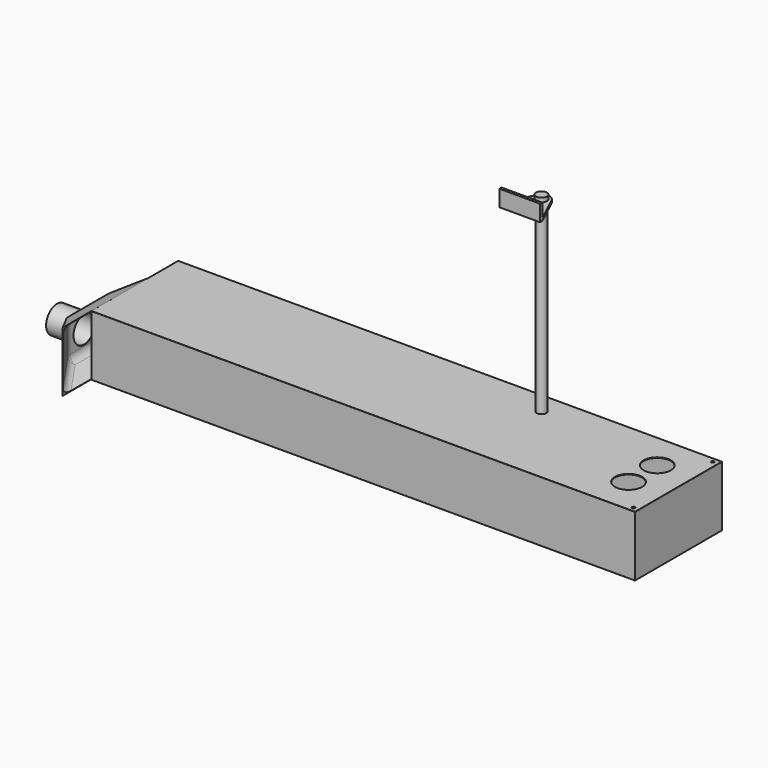
from build123d import *

# Parameters (mm, degrees)
F0_W      = 2000
F0_H      = 400
F1_DEPTH  = 220
F4_W      = 2000
F4_H      = 400
F4_R      = 6
F4_R_2    = 5.5
F5_DEPTH  = 3
F6_T      = 2.5
F7_R      = 1
F8_W      = 398
F8_H      = 221
F10_W     = 150
F10_H     = 150
F13_W     = 394
F13_H     = 217
F14_DEPTH = 5
F15_R     = 50
F16_DEPTH = 100
F17_T     = -1
F22_R     = 5
F23_DEPTH = 2.5
F26_R     = 17.5
F27_DEPTH = 10
F28_W     = 150
F28_H     = 10
F29_DEPTH = 50
F30_R     = 17.5
F31_DEPTH = 700
F33_R     = 17.5
F34_DEPTH = 10
F35_W     = 150
F35_H     = 10
F36_DEPTH = 50
F37_R     = 20
F38_DEPTH = 15
F39_R     = 20
F40_DEPTH = 15
F41_R     = 30
F43_SIZE  = 1
F44_R     = 50
F45_DEPTH = 25


# Not quite as in the source:
# - two fillets or chamfers of one size are made in one step
# - a shell that OpenCascade refuses in one call is made with other operations: the cavity is built on its own and cut out


with BuildPart() as f1:
    # F0 (on Top) → F1 (new body)
    with BuildSketch(Plane.XY):
        Rectangle(F0_W, F0_H)
    extrude(amount=F1_DEPTH)

    # F4 (on offset) → F5 (join, through all)
    with BuildSketch(Plane.XY.offset(223)):
        Rectangle(F4_W, F4_H)
        with Locations((980, -182)):
            Circle(F4_R, mode=Mode.SUBTRACT)
        with Locations((980, 182)):
            Circle(F4_R, mode=Mode.SUBTRACT)
        with Locations((980, -182)):
            Circle(F4_R)
        with Locations((980, -182)):
            Circle(F4_R_2, mode=Mode.SUBTRACT)
        with Locations((980, 182)):
            Circle(F4_R)
        with Locations((980, 182)):
            Circle(F4_R_2, mode=Mode.SUBTRACT)
    extrude(amount=-F5_DEPTH)

    # F6: shell of thickness 2.5, made by hand


with BuildPart() as f6_core1:
    # F6_t2: copy of F1
    add(f1.part)

    # the walls: a layer under each face that stays
    f6_faces = [f6_core1.faces().sort_by_distance(p)[0] for p in [
        (0, 200, 111.5),
        (0, 0, 0),
        (0, -200, 111.5),
        (-1000, 0, 111.5),
        (0, 0, 223),
        (974.5, 182, 221.5),
        (974.5, -182, 221.5),
        (1000, 0, 111.5),
    ]]
    thicken(f6_faces, amount=-F6_T, mode=Mode.SUBTRACT)


with BuildPart() as f1_1:
    add(f1.part)

    # what is left inside the walls is the cavity
    f6_cavity = [f6_core1.part.solids().sort_by_distance(p)[0] for p in [
        (0, -65.833333, 2.525),
    ]]
    add(f6_cavity, mode=Mode.SUBTRACT)

    # F7
    f7_edges = [f1_1.edges().sort_by_distance(p)[0] for p in [
        (0, -200, 223),
        (0, 200, 223),
        (0, -200, 0),
        (0, 200, 0),
        (1000, 0, 0),
        (1000, -200, 111.5),
        (1000, 0, 223),
        (1000, 200, 111.5),
        (-1000, 0, 0),
        (-1000, -200, 111.5),
        (-1000, 0, 223),
        (-1000, 200, 111.5),
    ]]
    fillet(f7_edges, radius=F7_R)

    # F13 (on face) → F14 (cut)
    with BuildSketch(Plane(origin=(-1000, 0, 0), x_dir=(0, -1, 0), z_dir=(-1, 0, 0))):
        with Locations((0, 111.5)):
            Rectangle(F13_W, F13_H)
    extrude(amount=-F14_DEPTH, mode=Mode.SUBTRACT)

    # F22 (on face) → F23 (join, through all)
    with BuildSketch(Plane(origin=(0, 0, 0), x_dir=(1, 0, 0), z_dir=(0, 0, -1))):
        with Locations((-950, 0)):
            Circle(F22_R)
        with Locations((950, 0)):
            Circle(F22_R)
    extrude(amount=-F23_DEPTH)

    # F44 (on face) → F45 (cut)
    with BuildSketch(Plane.XY.offset(223)):
        with Locations((869, 66)):
            Circle(F44_R)
        with Locations((869, -66)):
            Circle(F44_R)
    extrude(amount=-F45_DEPTH, mode=Mode.SUBTRACT)


with BuildPart() as f11:
    # F8 (on face) → F11 section 0
    with BuildSketch(Plane(origin=(-1000, 0, 0), x_dir=(0, -1, 0), z_dir=(-1, 0, 0))):
        with Locations((0, 111.5)):
            Rectangle(F8_W, F8_H)
    # F10 (on offset) → F11 section 1
    with BuildSketch(Plane(origin=(-1080, 0, 0), x_dir=(0, -1, 0), z_dir=(-1, 0, 0))):
        with Locations((0, 110)):
            Rectangle(F10_W, F10_H)
    loft()


with BuildPart() as f11_1:
    # F12: moved
    add(f11.part.moved(Location((0, -132, 0))))

    # F15 (on face) → F16 (join)
    with BuildSketch(Plane(origin=(-1080, 0, 0), x_dir=(0, -1, 0), z_dir=(-1, 0, 0))):
        with Locations((132, 110)):
            Circle(F15_R)
    extrude(amount=F16_DEPTH)

    # F17
    f17_openings = [f11_1.faces().sort_by_distance(p)[0] for p in [
        (-1180, -132, 110),
        (-1000, -132, 111.5),
    ]]
    offset(amount=F17_T, openings=f17_openings, kind=Kind.INTERSECTION)

    # F41
    f41_edges = [f11_1.edges().sort_by_distance(p)[0] for p in [
        (-1080, -207, 110),
        (-1080, -132, 185),
        (-1080, -132, 35),
        (-1080, -57, 110),
        (-1039.5, -267.930413, 202.629476),
        (-1079, -206.705413, 110.011146),
        (-1039.5, -267.930414, 18.874066),
        (-1039.5, 3.930413, 202.629476),
        (-1079, -132, 184.360726),
        (-1079, -131.999939, 35.661566),
        (-1079, -57.294587, 110.011119),
        (-1039.5, 3.930413, 18.874066),
    ]]
    fillet(f41_edges, radius=F41_R)

    # F43
    f43_edges = [f11_1.edges().sort_by_distance(p)[0] for p in [
        (-1079, -83, 110),
    ]]
    chamfer(f43_edges, length=F43_SIZE)


with BuildPart() as f27:
    # F26 (on line) → F27 (new body)
    with BuildSketch(Plane.XY.offset(200)):
        with BuildLine():
            Line((475, 20), (475, 30))
            Line((475, 30), (427.1288558138, 132.66))
            ThreePointArc((427.1288558138, 132.66), (400, 149.8527683618), (372.8711441862, 132.66))
            Line((372.8711441862, 132.66), (325, 30))
            Line((325, 30), (325, 20))
            Line((325, 20), (475, 20))
        make_face()
        with Locations((400, 119.8527683618)):
            Circle(F26_R, mode=Mode.SUBTRACT)
    extrude(amount=-F27_DEPTH)

    # F28 (on face) → F29 (join)
    with BuildSketch(Plane(origin=(0, 0, 190), x_dir=(1, 0, 0), z_dir=(0, 0, -1))):
        with Locations((400, -25)):
            Rectangle(F28_W, F28_H)
    extrude(amount=F29_DEPTH)


with BuildPart() as f31:
    # F30 (on face) → F31 (new body)
    with BuildSketch(Plane.XY.offset(200)):
        with Locations((400, 119.8527683618)):
            Circle(F30_R)
    extrude(amount=F31_DEPTH)


with BuildPart() as f34:
    # F33 (on offset) → F34 (new body)
    with BuildSketch(Plane.XY.offset(900)):
        with BuildLine():
            Line((475, 30), (427.1288558138, 132.66))
            ThreePointArc((427.1288558138, 132.66), (400, 149.8527683618), (372.8711441862, 132.66))
            Line((372.8711441862, 132.66), (325, 30))
            Line((325, 30), (325, 20))
            Line((325, 20), (475, 20))
            Line((475, 20), (475, 30))
        make_face()
        with Locations((400, 119.8527683618)):
            Circle(F33_R, mode=Mode.SUBTRACT)
    extrude(amount=F34_DEPTH)

    # F35 (on face) → F36 (join)
    with BuildSketch(Plane.XY.offset(910)):
        with Locations((400, 25)):
            Rectangle(F35_W, F35_H)
    extrude(amount=F36_DEPTH)


with BuildPart() as f38:
    # F37 (on face) → F38 (new body)
    with BuildSketch(Plane.XY.offset(910)):
        with Locations((400, 119.8527683618)):
            Circle(F37_R)
    extrude(amount=F38_DEPTH)


with BuildPart() as f40:
    # F39 (on face) → F40 (new body)
    with BuildSketch(Plane(origin=(0, 0, 190), x_dir=(1, 0, 0), z_dir=(0, 0, -1))):
        with Locations((400, -119.8527683618)):
            Circle(F39_R)
    extrude(amount=F40_DEPTH)


solid = Compound([f1_1.part, f11_1.part, f27.part, f31.part, f34.part, f38.part, f40.part])
